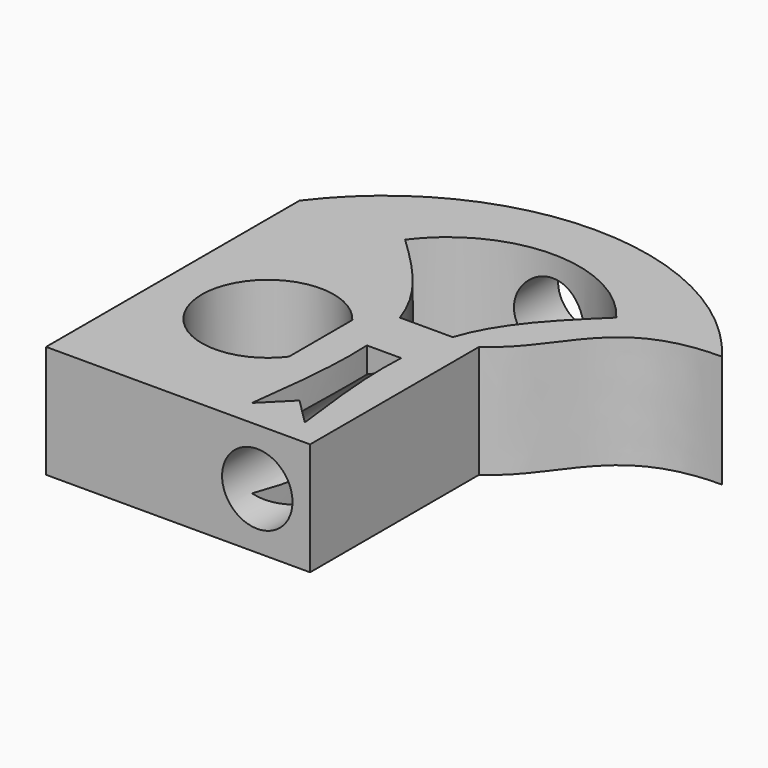
from build123d import *

# Parameters (mm, degrees)
F0_W          = 75
F0_H          = 75
F1_DEPTH      = 10
F1_DEPTH_BACK = 10
F3_DEPTH      = 20
F4_R          = 6.25
F5_DEPTH      = 75


# Not quite as in the source:
# - a feature names something its author has since deleted; it is built from what else it names


with BuildPart() as f1:
    # F0 (on Top) → F1 (new body, two sides)
    with BuildSketch(Plane.XY) as f1_sk:
        Rectangle(F0_W, F0_H)
    extrude(amount=F1_DEPTH)
    extrude(f1_sk.sketch, amount=-F1_DEPTH_BACK)

    # F2 (on face) → F3 (cut)
    with BuildSketch(Plane.XY.offset(10)):
        with BuildLine():
            Line((37.5, -37.5), (37.5, 18.75))
            add(Edge.make_bspline(
                [(9.375, 0), (18.75, 6.25), (18.75, 18.75), (37.5, 18.75)],
                knots=[0, 0, 0, 0, 33.8020432075, 33.8020432075, 33.8020432075, 33.8020432075], degree=3))
            Line((9.375, 0), (9.375, -37.5))
            Line((9.375, -37.5), (18.75, -37.5))
            Line((18.75, -37.5), (37.5, -37.5))
        make_face()
        with BuildLine():
            ThreePointArc((0, 37.5), (20.9631372891, 32.5512745781), (37.5, 18.75))
            Line((37.5, 18.75), (37.5, 37.5))
            Line((37.5, 37.5), (0, 37.5))
        make_face()
        with BuildLine():
            ThreePointArc((-37.5, 18.75), (-20.9631372891, 32.5512745781), (0, 37.5))
            Line((0, 37.5), (-37.5, 37.5))
            Line((-37.5, 37.5), (-37.5, 18.75))
        make_face()
        with BuildLine():
            Line((0, -28.125), (4.6875, -32.8125))
            add(Edge.make_bspline(
                [(4.6875, -32.8125), (3.6620711894, -24.6951237234), (2.6366423788, -16.5777474468), (3.0432450075, -9.375)],
                knots=[0, 0, 0, 0, 0.3697687561, 0.3697687561, 0.3697687561, 0.3697687561], degree=3))
            Line((3.0432450075, -9.375), (-3.0432450075, -9.375))
            add(Edge.make_bspline(
                [(-4.6875, -32.8125), (-3.6620711894, -24.6951237234), (-2.6366423788, -16.5777474468), (-3.0432450075, -9.375)],
                knots=[0, 0, 0, 0, 0.3697687561, 0.3697687561, 0.3697687561, 0.3697687561], degree=3))
            Line((-4.6875, -32.8125), (0, -28.125))
        make_face()
        with BuildLine():
            Line((-9.375, -18.75), (-9.375, -4.6875))
            ThreePointArc((-9.375, -4.6875), (-25.78125, -2.34375), (-28.125, -18.75))
            ThreePointArc((-28.125, -18.75), (-18.75, -23.4375), (-9.375, -18.75))
        make_face()
        with BuildLine():
            Line((-4.6875, 0), (4.6875, 0))
            add(Edge.make_bspline(
                [(4.6875, 0), (7.2279380084, 7.6213140251), (12.9889690042, 13.1856570125), (18.75, 18.75)],
                knots=[0.5419601085, 0.5419601085, 0.5419601085, 0.5419601085, 1, 1, 1, 1], degree=3))
            ThreePointArc((18.75, 18.75), (0, 28.1290022772), (-18.75, 18.75))
            add(Edge.make_bspline(
                [(-4.6875, 0), (-7.2279380084, 7.6213140251), (-12.9889690042, 13.1856570125), (-18.75, 18.75)],
                knots=[0.5419601085, 0.5419601085, 0.5419601085, 0.5419601085, 1, 1, 1, 1], degree=3))
        make_face()
    extrude(amount=-F3_DEPTH, mode=Mode.SUBTRACT)

    # F4 (on face) → F5 (cut)
    with BuildSketch(Plane.XZ.offset(37.5)):
        Circle(F4_R)
    extrude(amount=-F5_DEPTH, mode=Mode.SUBTRACT)


solid = f1.part
